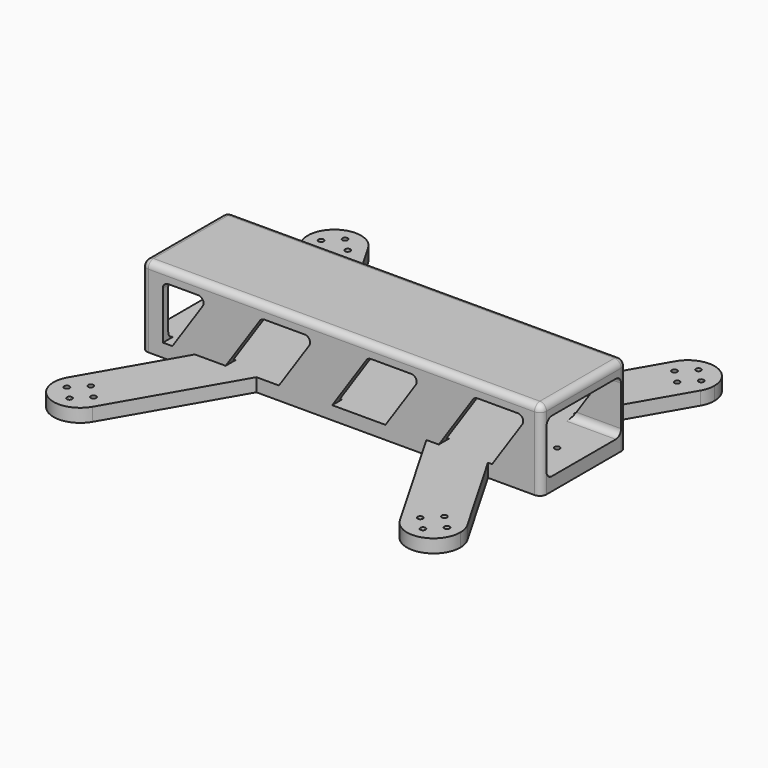
from build123d import *

# Parameters (mm, degrees)
F1_DEPTH  = 30
F2_W      = 165.0929152966
F2_H      = 57.5539949536
F2_W_2    = 169.7465479374
F2_H_2    = 58.0100673437
F3_DEPTH  = 25
F5_DEPTH  = 151.3407459622
F7_DEPTH  = 89.6420161514
F8_R      = 2.49999
F9_R      = 1
F10_DEPTH = 5.001
F11_R     = 1
F12_DEPTH = 5


# Not quite as in the source:
# - a fillet or chamfer is up to 0.001 mm smaller than in the source, because OpenCascade refuses the exact size


with BuildPart() as f1:
    # F0 (on Top) → F1 (new body)
    with BuildSketch(Plane.XY):
        Polygon((75, -20), (75, 20), (55, 20), (31.9059892324, 20), (-31.9059892324, 20), (-55, 20), (-75, 20), (-75, -20), (-55, -20), (-31.9059892324, -20), (31.9059892324, -20), (55, -20), align=None)
        with BuildLine():
            Line((31.9059892324, 20), (55, 20))
            Line((55, 20), (75, 54.6410161514))
            ThreePointArc((75, 54.6410161514), (61.3397459622, 50.9807621135), (57.6794919243, 64.6410161514))
            Line((57.6794919243, 64.6410161514), (31.9059892324, 20))
        make_face()
        with BuildLine():
            ThreePointArc((57.6794919243, 64.6410161514), (61.3397459622, 50.9807621135), (75, 54.6410161514))
            Line((75, 54.6410161514), (57.6794919243, 64.6410161514))
        make_face()
        with BuildLine():
            Line((57.6794919243, 64.6410161514), (75, 54.6410161514))
            ThreePointArc((75, 54.6410161514), (75.999004225, 57.0528257004), (76.3397459622, 59.6410161514))
            ThreePointArc((76.3397459622, 59.6410161514), (68.9279364132, 69.3002744143), (57.6794919243, 64.6410161514))
        make_face()
        with BuildLine():
            Line((75, -54.6410161514), (55, -20))
            Line((55, -20), (31.9059892324, -20))
            Line((31.9059892324, -20), (57.6794919243, -64.6410161514))
            ThreePointArc((57.6794919243, -64.6410161514), (61.3397459622, -50.9807621135), (75, -54.6410161514))
        make_face()
        with BuildLine():
            Line((-55, 20), (-31.9059892324, 20))
            Line((-31.9059892324, 20), (-57.6794919243, 64.6410161514))
            ThreePointArc((-57.6794919243, 64.6410161514), (-56.6804876993, 62.2292066024), (-56.3397459622, 59.6410161514))
            ThreePointArc((-56.3397459622, 59.6410161514), (-63.7515555111, 49.9817578885), (-75, 54.6410161514))
            Line((-75, 54.6410161514), (-55, 20))
        make_face()
        with BuildLine():
            ThreePointArc((76.3397459622, -59.6410161514), (75.999004225, -57.0528257004), (75, -54.6410161514))
            Line((75, -54.6410161514), (57.6794919243, -64.6410161514))
            ThreePointArc((57.6794919243, -64.6410161514), (68.9279364132, -69.3002744143), (76.3397459622, -59.6410161514))
        make_face()
        with BuildLine():
            Line((57.6794919243, -64.6410161514), (75, -54.6410161514))
            ThreePointArc((75, -54.6410161514), (61.3397459622, -50.9807621135), (57.6794919243, -64.6410161514))
        make_face()
        with BuildLine():
            ThreePointArc((-56.3397459622, 59.6410161514), (-56.6804876993, 62.2292066024), (-57.6794919243, 64.6410161514))
            Line((-57.6794919243, 64.6410161514), (-75, 54.6410161514))
            ThreePointArc((-75, 54.6410161514), (-63.7515555111, 49.9817578885), (-56.3397459622, 59.6410161514))
        make_face()
        with BuildLine():
            Line((-75, 54.6410161514), (-57.6794919243, 64.6410161514))
            ThreePointArc((-57.6794919243, 64.6410161514), (-71.3397459622, 68.3012701892), (-75, 54.6410161514))
        make_face()
        with BuildLine():
            Line((-57.6794919243, -64.6410161514), (-31.9059892324, -20))
            Line((-31.9059892324, -20), (-55, -20))
            Line((-55, -20), (-75, -54.6410161514))
            ThreePointArc((-75, -54.6410161514), (-63.7515555111, -49.9817578885), (-56.3397459622, -59.6410161514))
            ThreePointArc((-56.3397459622, -59.6410161514), (-56.6804876993, -62.2292066024), (-57.6794919243, -64.6410161514))
        make_face()
        with BuildLine():
            ThreePointArc((-75, -54.6410161514), (-71.3397459622, -68.3012701892), (-57.6794919243, -64.6410161514))
            Line((-57.6794919243, -64.6410161514), (-75, -54.6410161514))
        make_face()
        with BuildLine():
            Line((-75, -54.6410161514), (-57.6794919243, -64.6410161514))
            ThreePointArc((-57.6794919243, -64.6410161514), (-56.6804876993, -62.2292066024), (-56.3397459622, -59.6410161514))
            ThreePointArc((-56.3397459622, -59.6410161514), (-63.7515555111, -49.9817578885), (-75, -54.6410161514))
        make_face()
    extrude(amount=F1_DEPTH)

    # F2 (on face) → F3 (cut)
    with BuildSketch(Plane.XY.offset(30)):
        with Locations((-4.5224651694, 48.7769974768)):
            Rectangle(F2_W, F2_H)
        with Locations((-0.866048038, -49.0050336719)):
            Rectangle(F2_W_2, F2_H_2)
    extrude(amount=-F3_DEPTH, mode=Mode.SUBTRACT)

    # F4 (on face) → F5 (cut, through all)
    with BuildSketch(Plane(origin=(-75, 0, 0), x_dir=(0, -1, 0), z_dir=(-1, 0, 0))):
        with BuildLine():
            ThreePointArc((-17.5, 7.5), (-16.767766953, 5.732233047), (-15, 5))
            Line((-15, 5), (15, 5))
            ThreePointArc((15, 5), (16.767766953, 5.732233047), (17.5, 7.5))
            Line((17.5, 7.5), (17.5, 22.5))
            ThreePointArc((17.5, 22.5), (16.767766953, 24.267766953), (15, 25))
            Line((15, 25), (-15, 25))
            ThreePointArc((-15, 25), (-16.767766953, 24.267766953), (-17.5, 22.5))
            Line((-17.5, 22.5), (-17.5, 7.5))
        make_face()
    extrude(amount=-F5_DEPTH, mode=Mode.SUBTRACT)

    # F6 (on face) → F7 (cut, through all)
    with BuildSketch(Plane.XZ.offset(20)):
        with BuildLine():
            ThreePointArc((67.9038453252, 21.883735206), (68.0096360455, 23.9400719153), (66.2443415109, 25))
            Line((66.2443415109, 25), (51.0650595659, 25))
            ThreePointArc((51.0650595659, 25), (50.1249876505, 24.7652945346), (49.4055557516, 24.116264794))
            Line((49.4055557516, 24.116264794), (36.5470053838, 5))
            Line((36.5470053838, 5), (56.5470053838, 5))
            Line((56.5470053838, 5), (67.9038453252, 21.883735206))
        make_face()
        with BuildLine():
            ThreePointArc((-65, 25), (-66.4142135624, 24.4142135624), (-67, 23))
            Line((-67, 23), (-67, 5))
            Line((-67, 5), (-63.4529946162, 5))
            Line((-63.4529946162, 5), (-52.0961546748, 21.883735206))
            ThreePointArc((-52.0961546748, 21.883735206), (-51.9903639545, 23.9400719153), (-53.7556584891, 25))
            Line((-53.7556584891, 25), (-65, 25))
        make_face()
        with BuildLine():
            ThreePointArc((-28.9349404341, 25), (-29.8750123495, 24.7652945346), (-30.5944442484, 24.116264794))
            Line((-30.5944442484, 24.116264794), (-43.4529946162, 5))
            Line((-43.4529946162, 5), (-23.4529946162, 5))
            Line((-23.4529946162, 5), (-12.0961546748, 21.883735206))
            ThreePointArc((-12.0961546748, 21.883735206), (-11.9903639545, 23.9400719153), (-13.7556584891, 25))
            Line((-13.7556584891, 25), (-28.9349404341, 25))
        make_face()
        with BuildLine():
            ThreePointArc((11.0650595659, 25), (10.1249876505, 24.7652945346), (9.4055557516, 24.116264794))
            Line((9.4055557516, 24.116264794), (-3.4529946162, 5))
            Line((-3.4529946162, 5), (16.5470053838, 5))
            Line((16.5470053838, 5), (27.9038453252, 21.883735206))
            ThreePointArc((27.9038453252, 21.883735206), (28.0096360455, 23.9400719153), (26.2443415109, 25))
            Line((26.2443415109, 25), (11.0650595659, 25))
        make_face()
    extrude(amount=-F7_DEPTH, mode=Mode.SUBTRACT)

    # F8 (radius 2.5 in the source; OpenCascade refuses exactly that, so slightly less here)
    f8_edges = [f1.edges().sort_by_distance(p)[0] for p in [
        (-75, -20, 15),
        (0, -20, 30),
        (-75, 0, 30),
        (-75, 20, 15),
        (0, 20, 30),
        (75, 0, 30),
        (75, -20, 15),
        (75, 20, 15),
    ]]
    fillet(f8_edges, radius=F8_R)

    # F9 (on face) → F10 (cut, through all)
    with BuildSketch(Plane.XY.offset(5)):
        with Locations((-66.3397459622, 54.6410161514)):
            Circle(F9_R)
        with Locations((-66.3397459622, 64.6410161514)):
            Circle(F9_R)
        with Locations((66.3397459622, 64.6410161514)):
            Circle(F9_R)
        with Locations((66.3397459622, 54.6410161514)):
            Circle(F9_R)
        with Locations((-66.3397459622, -54.6410161514)):
            Circle(F9_R)
        with Locations((-66.3397459622, -64.6410161514)):
            Circle(F9_R)
        with Locations((-71.3397459622, 59.6410161514)):
            Circle(F9_R)
        with Locations((-61.3397459622, 59.6410161514)):
            Circle(F9_R)
        with Locations((71.3397459622, 59.6410161514)):
            Circle(F9_R)
        with Locations((61.3397459622, 59.6410161514)):
            Circle(F9_R)
        with Locations((-61.3397459622, -59.6410161514)):
            Circle(F9_R)
        with Locations((-71.3397459622, -59.6410161514)):
            Circle(F9_R)
        with Locations((66.3397459622, -54.6410161514)):
            Circle(F9_R)
        with Locations((66.3397459622, -64.6410161514)):
            Circle(F9_R)
        with Locations((71.3397459622, -59.6410161514)):
            Circle(F9_R)
        with Locations((61.3397459622, -59.6410161514)):
            Circle(F9_R)
    extrude(amount=-F10_DEPTH, mode=Mode.SUBTRACT)

    # F11 (on face) → F12 (cut)
    with BuildSketch(Plane(origin=(0, 0, 0), x_dir=(1, 0, 0), z_dir=(0, 0, -1))):
        with Locations((-65, 0)):
            Circle(F11_R)
        with Locations((65, 0)):
            Circle(F11_R)
    extrude(amount=-F12_DEPTH, mode=Mode.SUBTRACT)


solid = f1.part
